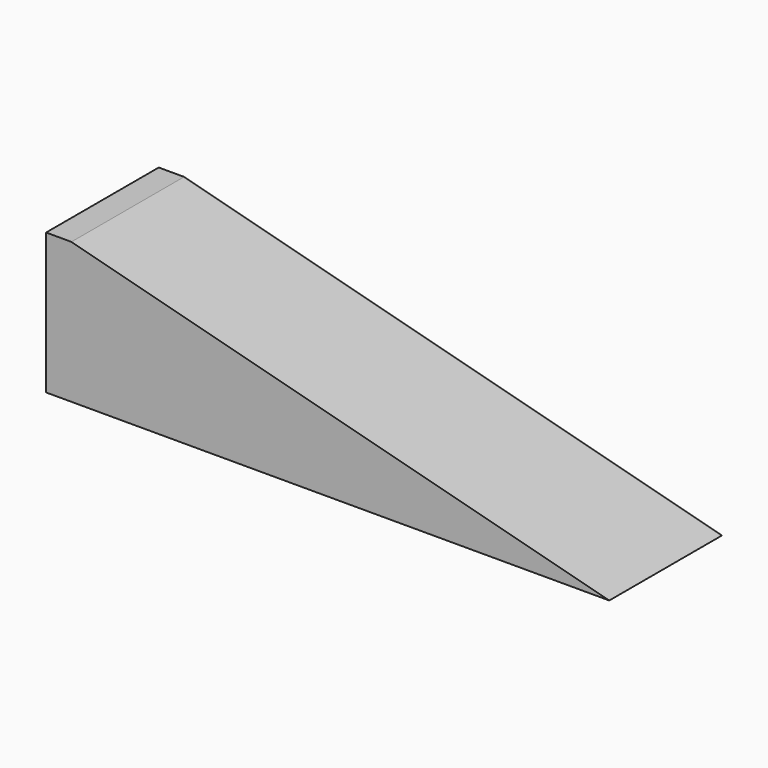
from build123d import *

# Parameters (mm, degrees)
F0_W     = 20
F0_H     = 5
F1_DEPTH = 5
F2_SIZE2 = 4.99999
F2_SIZE  = 19.09999


# Not quite as in the source:
# - a fillet or chamfer is up to 0.001 mm smaller than in the source, because OpenCascade refuses the exact size


with BuildPart() as f1:
    # F0 (on Top) → F1 (new body)
    with BuildSketch(Plane.XY):
        Rectangle(F0_W, F0_H)
    extrude(amount=F1_DEPTH)

    # F2 (size 19.1 and 5 in the source; OpenCascade refuses exactly that, so slightly less here)
    f2_edges = [f1.edges().sort_by_distance(p)[0] for p in [
        (10, 0, 5),
    ]]
    f2_side = f1.faces().sort_by_distance((0, 0, 5))[0]
    chamfer(f2_edges, length=F2_SIZE, length2=F2_SIZE2, reference=f2_side)


solid = f1.part
